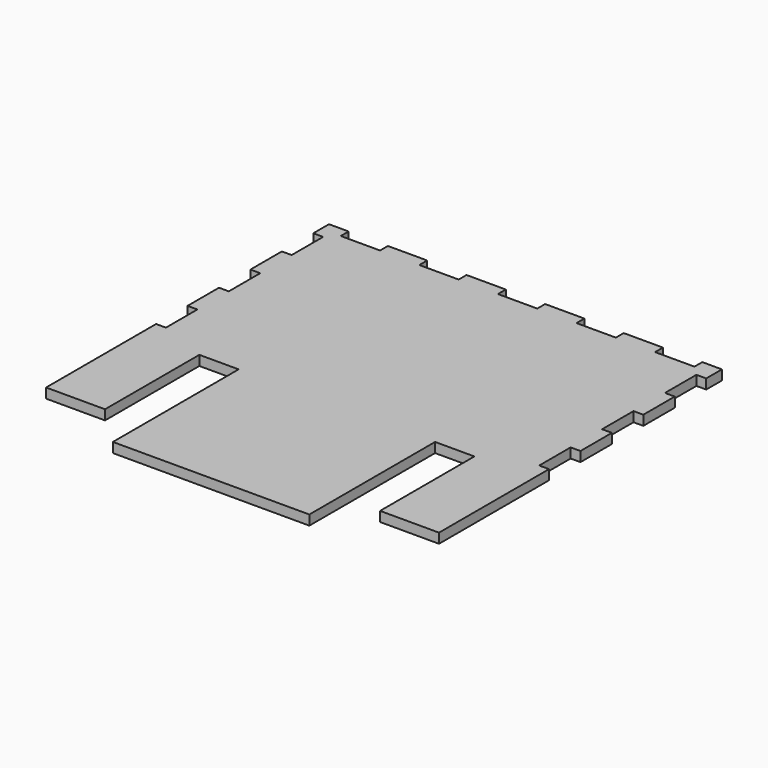
from build123d import *

# Parameters (mm, degrees)
F0_W     = 31.75
F0_H     = 50.8
F0_W_2   = 3.175
F0_H_2   = 12.7
F0_W_3   = 12.7
F0_H_3   = 3.175
F0_W_4   = 19.05
F0_H_4   = 38.1
F1_DEPTH = 3.175


# Not quite as in the source:
# - a feature names something its author has since deleted; it is built from what else it names


with BuildPart() as f1:
    # F0 (on Top) → F1 (new body)
    with BuildSketch(Plane.XY):
        with Locations((-8.6727611423, -50.1471598029)):
            Rectangle(F0_W, F0_H)
        with Locations((-40.4227611423, -50.1471598029)):
            Rectangle(F0_W, F0_H)
        Polygon((-81.6977611423, 51.4528401971), (-88.0477611423, 51.4528401971), (-88.0477611423, 45.1028401971), (-84.8727611423, 45.1028401971), (-84.8727611423, 32.4028401971), (-84.8727611423, 19.7028401971), (-84.8727611423, 7.0028401971), (-84.8727611423, -5.6971598029), (-84.8727611423, -18.3971598029), (-88.0477611423, -18.3971598029), (-88.0477611423, -24.7471598029), (-68.9977611423, -24.7471598029), (-56.2977611423, -24.7471598029), (-24.5477611423, -24.7471598029), (7.2022388577, -24.7471598029), (19.9022388577, -24.7471598029), (38.9522388577, -24.7471598029), (38.9522388577, -18.3971598029), (35.7772388577, -18.3971598029), (35.7772388577, -5.6971598029), (35.7772388577, 7.0028401971), (35.7772388577, 19.7028401971), (35.7772388577, 32.4028401971), (35.7772388577, 45.1028401971), (38.9522388577, 45.1028401971), (38.9522388577, 51.4528401971), (32.6022388577, 51.4528401971), (32.6022388577, 48.2778401971), (19.9022388577, 48.2778401971), (7.2022388577, 48.2778401971), (-5.4977611423, 48.2778401971), (-18.1977611423, 48.2778401971), (-30.8977611423, 48.2778401971), (-43.5977611423, 48.2778401971), (-56.2977611423, 48.2778401971), (-68.9977611423, 48.2778401971), (-81.6977611423, 48.2778401971), align=None)
        with Locations((-86.4602611423, 26.0528401971)):
            Rectangle(F0_W_2, F0_H_2)
        with Locations((-86.4602611423, 0.6528401971)):
            Rectangle(F0_W_2, F0_H_2)
        with Locations((37.3647388577, 0.6528401971)):
            Rectangle(F0_W_2, F0_H_2)
        with Locations((37.3647388577, 26.0528401971)):
            Rectangle(F0_W_2, F0_H_2)
        with Locations((-62.6477611423, 49.8653401971)):
            Rectangle(F0_W_3, F0_H_3)
        with Locations((-11.8477611423, 49.8653401971)):
            Rectangle(F0_W_3, F0_H_3)
        with Locations((-37.2477611423, 49.8653401971)):
            Rectangle(F0_W_3, F0_H_3)
        with Locations((-78.5227611423, -43.7971598029)):
            Rectangle(F0_W_4, F0_H_4)
        with Locations((29.4272388577, -43.7971598029)):
            Rectangle(F0_W_4, F0_H_4)
        with Locations((13.5522388577, 49.8653401971)):
            Rectangle(F0_W_3, F0_H_3)
    extrude(amount=F1_DEPTH)


solid = f1.part
